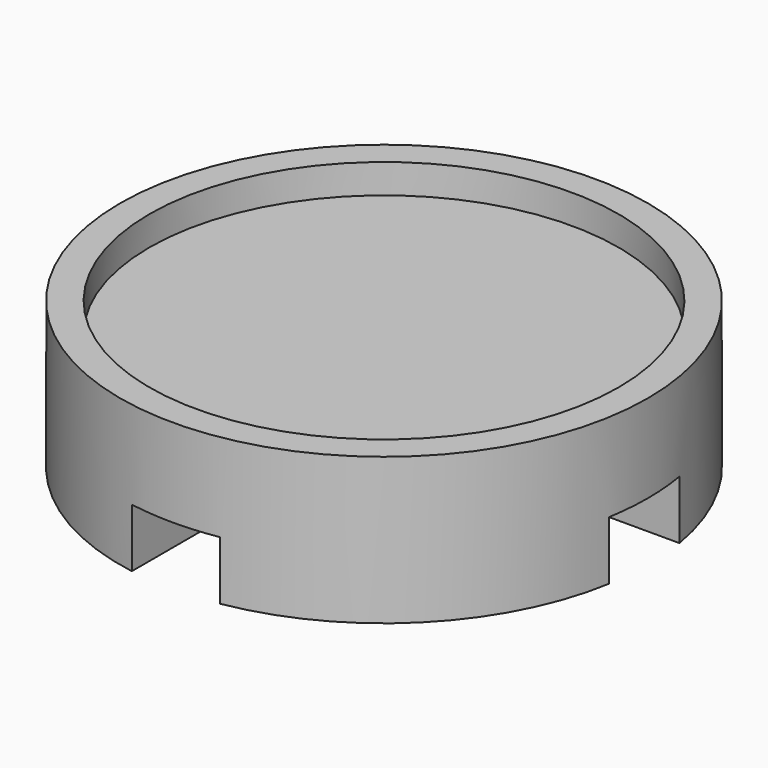
from build123d import *

# Parameters (mm, degrees)
F0_R     = 9
F1_DEPTH = 4
F3_W     = 3
F3_H     = 3
F4_DEPTH = 2
F2_R     = 9
F2_R_2   = 8
F5_DEPTH = 1


# Not quite as in the source:
# - a feature names something its author has since deleted; it is built from what else it names


with BuildPart() as f1:
    # F0 (on Top) → F1 (new body)
    with BuildSketch(Plane.XY):
        with Locations((-31.3306450844, 19.7580661625)):
            Circle(F0_R)
    extrude(amount=F1_DEPTH)

    # F3 (on face) → F4 (cut)
    with BuildSketch(Plane(origin=(0, 0, 0), x_dir=(1, 0, 0), z_dir=(0, 0, -1))):
        with BuildLine():
            ThreePointArc((-32.8306450844, -28.6321858371), (-32.0832814269, -28.7265408676), (-31.3306450844, -28.7580661625))
            ThreePointArc((-31.3306450844, -28.7580661625), (-30.5780087419, -28.7265408676), (-29.8306450844, -28.6321858371))
            Line((-29.8306450844, -28.6321858371), (-29.8306450844, -21.2580661625))
            Line((-29.8306450844, -21.2580661625), (-32.8306450844, -21.2580661625))
            Line((-32.8306450844, -21.2580661625), (-32.8306450844, -28.6321858371))
        make_face()
        with BuildLine():
            ThreePointArc((-40.204764759, -18.2580661625), (-40.2991197895, -19.0054298199), (-40.3306450844, -19.7580661625))
            ThreePointArc((-40.3306450844, -19.7580661625), (-40.2991197895, -20.510702505), (-40.204764759, -21.2580661625))
            Line((-40.204764759, -21.2580661625), (-32.8306450844, -21.2580661625))
            Line((-32.8306450844, -21.2580661625), (-32.8306450844, -18.2580661625))
            Line((-32.8306450844, -18.2580661625), (-40.204764759, -18.2580661625))
        make_face()
        with Locations((-31.3306450844, -19.7580661625)):
            Rectangle(F3_W, F3_H)
        with BuildLine():
            Line((-29.8306450844, -18.2580661625), (-29.8306450844, -21.2580661625))
            Line((-29.8306450844, -21.2580661625), (-22.4565254097, -21.2580661625))
            ThreePointArc((-22.4565254097, -21.2580661625), (-22.3621703793, -20.510702505), (-22.3306450844, -19.7580661625))
            ThreePointArc((-22.3306450844, -19.7580661625), (-22.3621703793, -19.0054298199), (-22.4565254097, -18.2580661625))
            Line((-22.4565254097, -18.2580661625), (-29.8306450844, -18.2580661625))
        make_face()
        with BuildLine():
            Line((-32.8306450844, -10.8839464878), (-32.8306450844, -18.2580661625))
            Line((-32.8306450844, -18.2580661625), (-29.8306450844, -18.2580661625))
            Line((-29.8306450844, -18.2580661625), (-29.8306450844, -10.8839464878))
            ThreePointArc((-29.8306450844, -10.8839464878), (-30.5780087419, -10.7895914574), (-31.3306450844, -10.7580661625))
            ThreePointArc((-31.3306450844, -10.7580661625), (-32.0832814269, -10.7895914574), (-32.8306450844, -10.8839464878))
        make_face()
    extrude(amount=-F4_DEPTH, mode=Mode.SUBTRACT)

    # F2 (on face) → F5 (join)
    with BuildSketch(Plane.XY.offset(4)):
        with Locations((-31.3306450844, 19.7580661625)):
            Circle(F2_R)
        with Locations((-31.3306450844, 19.7580661625)):
            Circle(F2_R_2, mode=Mode.SUBTRACT)
    extrude(amount=F5_DEPTH)


solid = f1.part
